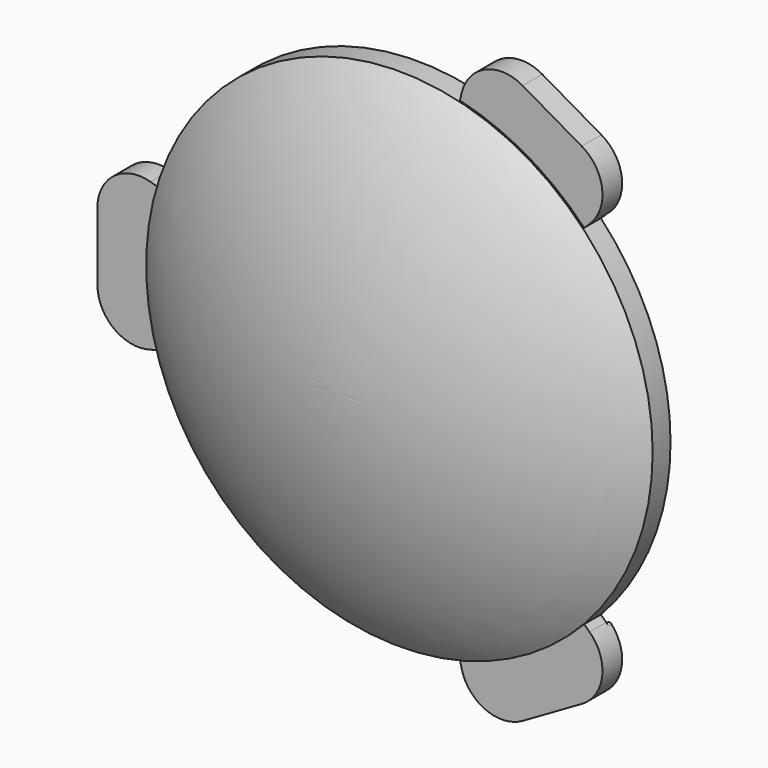
from build123d import *

# Parameters (mm, degrees)
F0_W          = 17
F0_H          = 1.5
F3_DEPTH      = 0.75
F3_DEPTH_BACK = 0.65
F4_DEPTH      = 1
F5_T1_DEPTH   = 0.7858762015
F6_COUNT      = 3
F6_ANGLE      = 240


# Not quite as in the source:
# - a fillet or chamfer that OpenCascade refuses, or shapes differently, is made with other operations: its cross-section is extruded or revolved along the edge and cut away or added
# - a feature names something its author has since deleted; it is built from what else it names


with BuildPart() as f1:
    # F0 (on Top) → F1 (revolve)
    with BuildSketch(Plane.XY):
        with BuildLine():
            Line((0, 2.9235986368), (0, 0.75))
            Line((0, 0.75), (17, 0.75))
            add(Edge.make_bspline(
                [(17, 0.75), (14.7452850491, 2.0917814691), (7.445672527, 2.9235986368), (0, 2.9235986368)],
                knots=[0, 0, 0, 0, 17.1383934788, 17.1383934788, 17.1383934788, 17.1383934788], degree=3))
        make_face()
        with Locations((8.5, 0)):
            Rectangle(F0_W, F0_H)
        with BuildLine():
            Line((17, -0.75), (0, -0.75))
            Line((0, -0.75), (0, -5.8664013632))
            add(Edge.make_bspline(
                [(17, -0.75), (13.8637118638, -3.1852589455), (7.4548930861, -5.8664013632), (0, -5.8664013632)],
                knots=[0, 0, 0, 0, 17.7532409128, 17.7532409128, 17.7532409128, 17.7532409128], degree=3))
        make_face()
    revolve(axis=Axis((0, 1.8367993184, 0), (0, 1, 0)))

    # F2 (on Front) → F3 (join, two sides)
    with BuildSketch(Plane.XZ) as f3_sk:
        with BuildLine():
            ThreePointArc((-16.7830230255, -4.9578360326), (-17.5, 0), (-16.7830230255, 4.9578360326))
            ThreePointArc((-16.7830230255, 4.9578360326), (-19.2347780947, 4.5186022412), (-20.3506106924, 2.2917329463))
            Line((-20.3506106924, 2.2917329463), (-20.3506106924, 0))
            Line((-20.3506106924, 0), (-20.3506106924, -2.2917329463))
            ThreePointArc((-20.3506106924, -2.2917329463), (-19.2347780947, -4.5186022412), (-16.7830230255, -4.9578360326))
        make_face()
        with BuildLine():
            ThreePointArc((-16.3035080819, -4.8161835745), (-17, 0), (-16.3035080819, 4.8161835745))
            Line((-16.3035080819, 4.8161835745), (-16.7830230255, 4.9578360326))
            ThreePointArc((-16.7830230255, 4.9578360326), (-17.5, 0), (-16.7830230255, -4.9578360326))
            Line((-16.7830230255, -4.9578360326), (-16.3035080819, -4.8161835745))
        make_face()
    extrude(amount=-F3_DEPTH)
    extrude(f3_sk.sketch, amount=F3_DEPTH_BACK)

    # F2 (on Front) → F4 (join)
    with BuildSketch(Plane.XZ):
        with BuildLine():
            ThreePointArc((-16.7830230255, -4.9578360326), (-17.5, 0), (-16.7830230255, 4.9578360326))
            ThreePointArc((-16.7830230255, 4.9578360326), (-19.2347780947, 4.5186022412), (-20.3506106924, 2.2917329463))
            Line((-20.3506106924, 2.2917329463), (-20.3506106924, 0))
            Line((-20.3506106924, 0), (-20.3506106924, -2.2917329463))
            ThreePointArc((-20.3506106924, -2.2917329463), (-19.2347780947, -4.5186022412), (-16.7830230255, -4.9578360326))
        make_face()
    extrude(amount=-F4_DEPTH)

    # F5: fillet of radius 0.2 on 2 edges, made by hand

    # F5_s2 → F5_t1 (cut)
    with BuildSketch(Plane.XZ.offset(-1.5358762015)):
        with BuildLine():
            ThreePointArc((-16.9907798648, -5.0105923048), (-16.8612192668, -4.9182617144), (-16.84003675, -4.7605842351))
            ThreePointArc((-16.84003675, -4.7605842351), (-16.8118191828, -4.8592937518), (-16.7830230255, -4.9578360326))
            ThreePointArc((-16.7830230255, -4.9578360326), (-16.8863927879, -4.9862172864), (-16.9907798648, -5.0105923048))
        make_face()
        with BuildLine():
            ThreePointArc((-16.9907798648, 5.0105923048), (-16.8612192668, 4.9182617144), (-16.84003675, 4.7605842351))
            ThreePointArc((-16.84003675, 4.7605842351), (-16.8118191828, 4.8592937518), (-16.7830230255, 4.9578360326))
            ThreePointArc((-16.7830230255, 4.9578360326), (-16.8863927879, 4.9862172864), (-16.9907798648, 5.0105923048))
        make_face()
    extrude(amount=F5_T1_DEPTH, mode=Mode.SUBTRACT)

    # F6: F1 ×3 about axis
    f6_axis = Axis((0, -3.3082006816, 0), (0, -1, 0))


with BuildPart() as f1_1:
    add(f1.part)
    for i in range(1, F6_COUNT):
        add(f1.part.rotate(f6_axis, i * F6_ANGLE / (F6_COUNT - 1)))


solid = f1_1.part
